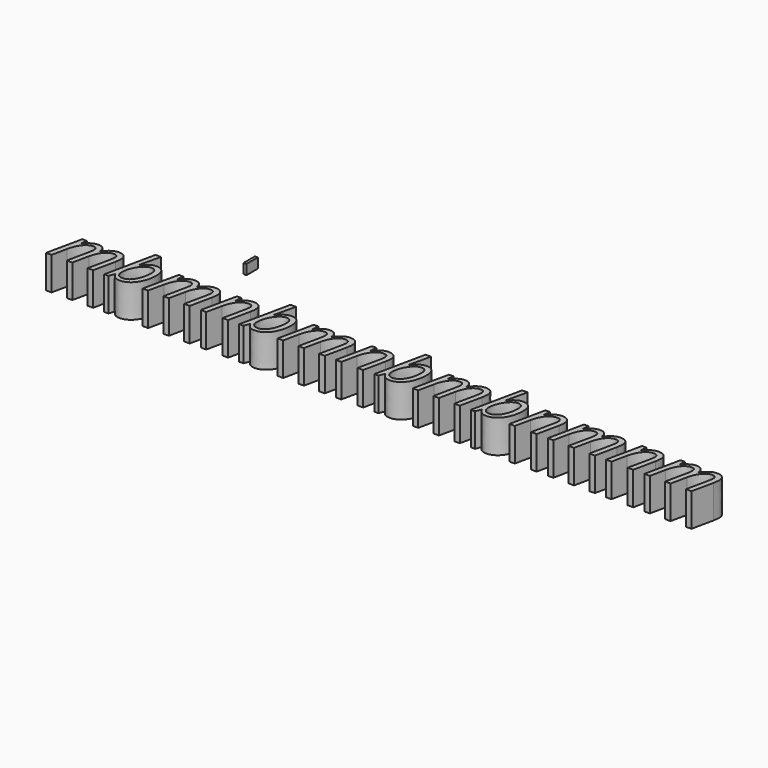
from build123d import *

# Parameters (mm, degrees)
F0_TEXT_SIZE = 167.1679305016
F1_DEPTH     = 83
F2_W         = 7.1457922459
F2_H         = 35.4455262423
F3_DEPTH     = 25


# Not quite as in the source:
# - Text() gives the source's letters only with a copy of the font that has no kerning and outlines rounded to 1/6400 em; it was checked with that copy


with BuildPart() as f1:
    # F0 (on Top) → F1 (new body)
    with BuildSketch(Plane.XY):
        with Locations((-169.9565649033, -111.1180186272)):
            Text('mbmnbmnbmbnmnm', F0_TEXT_SIZE, font='Open Sans', font_style=FontStyle.ITALIC, text_align=(TextAlign.LEFT, TextAlign.BOTTOM))
    extrude(amount=F1_DEPTH)


with BuildPart() as f3:
    # F2 (on Top) → F3 (new body)
    with BuildSketch(Plane.XY):
        with Locations((97.5247174501, 202.1742984653)):
            Rectangle(F2_W, F2_H)
    extrude(amount=F3_DEPTH)


solid = Compound([f1.part, f3.part])
